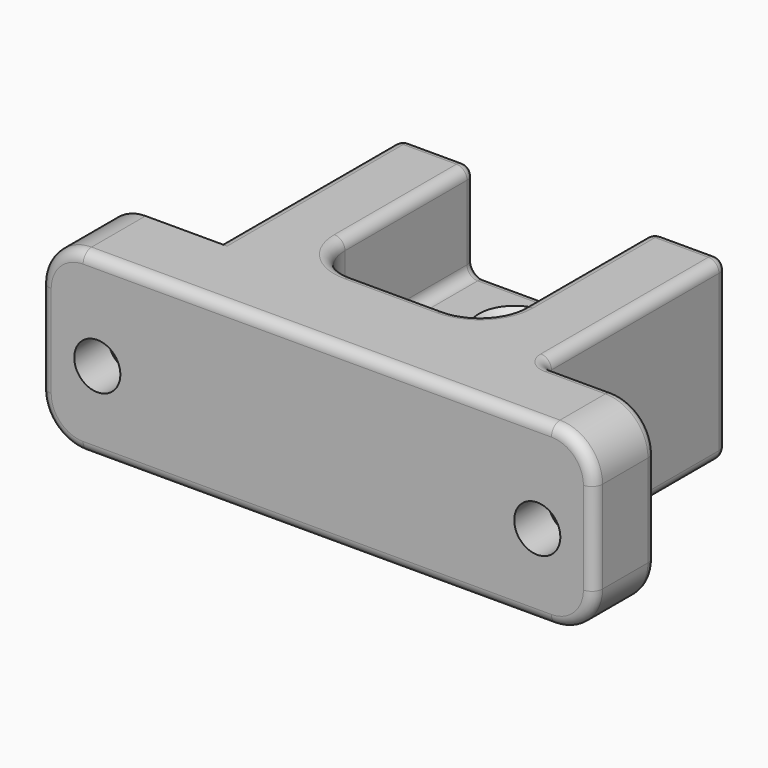
from build123d import *

# Parameters (mm, degrees)
F0_W           = 156
F0_H           = 50
F1_DEPTH       = 87
F2_W           = 32
F2_H           = 65
F3_DEPTH       = 50
F4_W           = 50
F4_H           = 58
F5_DEPTH       = 27
F7_D           = 13
F7_CBORE_D     = 18
F7_CBORE_DEPTH = 10
F9_D           = 13
F9_CSINK_D     = 20
F9_CSINK_ANGLE = 90
F10_R          = 12
F11_R          = 3


with BuildPart() as f1:
    # F0 (on Front) → F1 (new body)
    with BuildSketch(Plane.XZ):
        with Locations((78, 25)):
            Rectangle(F0_W, F0_H)
    extrude(amount=F1_DEPTH)

    # F2 (on face) → F3 (cut, through all)
    with BuildSketch(Plane.XY.offset(50)):
        with Locations((16, -32.5)):
            Rectangle(F2_W, F2_H)
        with Locations((140, -32.5)):
            Rectangle(F2_W, F2_H)
    extrude(amount=-F3_DEPTH, mode=Mode.SUBTRACT)

    # F4 (on face) → F5 (cut)
    with BuildSketch(Plane.XY.offset(50)):
        with Locations((78, -29)):
            Rectangle(F4_W, F4_H)
    extrude(amount=-F5_DEPTH, mode=Mode.SUBTRACT)

    # F7 (through all)
    with Locations(Plane(origin=(0, -65, 0), x_dir=(-1, 0, 0), z_dir=(0, 1, 0))):
        with Locations((-140, 23), (-16, 23)):
            CounterBoreHole(F7_D / 2, F7_CBORE_D / 2, F7_CBORE_DEPTH)

    # F9 (through all)
    with Locations(Plane.XY.offset(23)):
        with Locations((76, -15), (76, -42)):
            CounterSinkHole(F9_D / 2, F9_CSINK_D / 2, counter_sink_angle=F9_CSINK_ANGLE)

    # F10
    f10_edges = [f1.edges().sort_by_distance(p)[0] for p in [
        (156, -76, 50),
        (156, -76, 0),
        (0, -76, 50),
        (0, -76, 0),
        (103, -58, 36.5),
        (53, -58, 36.5),
    ]]
    fillet(f10_edges, radius=F10_R)

    # F11
    f11_edges = [f1.edges().sort_by_distance(p)[0] for p in [
        (78, -87, 50),
        (78, -58, 50),
        (53, -23, 50),
        (103, -23, 50),
        (56.514719, -54.485281, 50),
        (99.485281, -54.485281, 50),
        (124, -32.5, 50),
        (134, -65, 50),
        (124, -65, 25),
        (124, 0, 25),
        (78, 0, 23),
        (53, -23, 23),
        (56.514719, -54.485281, 23),
        (78, 0, 0),
        (32, 0, 25),
        (32, -32.5, 50),
        (78, -87, 0),
        (32, -32.5, 0),
        (113.5, 0, 50),
        (42.5, 0, 50),
        (124, -32.5, 0),
        (0, -87, 25),
        (3.514719, -87, 46.485281),
        (3.514719, -87, 3.514719),
        (152.485281, -87, 46.485281),
        (152.485281, -87, 3.514719),
        (156, -87, 25),
        (134, -65, 0),
        (152.485281, -65, 46.485281),
        (152.485281, -65, 3.514719),
        (156, -65, 25),
        (103, 0, 36.5),
        (103, -23, 23),
        (99.485281, -54.485281, 23),
        (53, 0, 36.5),
        (78, -58, 23),
    ]]
    fillet(f11_edges, radius=F11_R)


solid = f1.part
